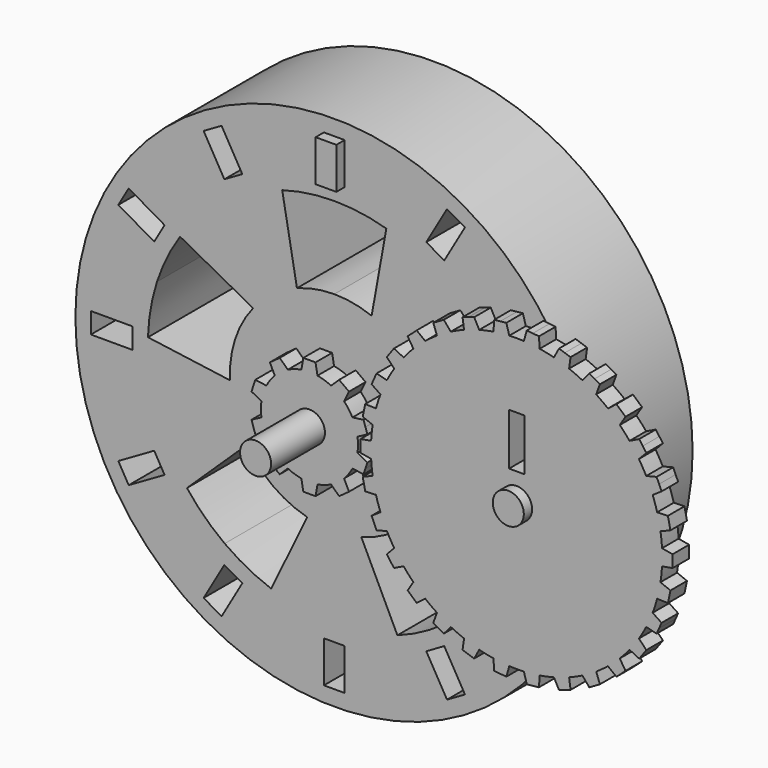
from build123d import *

# Parameters (mm, degrees)
F2_R      = 50
F3_DEPTH  = 24
F4_R      = 5
F4_R_2    = 3
F5_DEPTH  = 2
F6_DEPTH  = 19
F7_DEPTH  = 8
F12_DEPTH = 4
F14_DEPTH = 4
F15_W     = 4
F15_H     = 8
F15_W_2   = 8
F15_H_2   = 4
F16_DEPTH = 10
F17_DEPTH = 12
F19_DEPTH = 25
F20_W     = 3
F20_H     = 10
F21_DEPTH = 25


with BuildPart() as f3:
    # F2 (on Front) → F3 (new body)
    with BuildSketch(Plane.XZ):
        Circle(F2_R)
    extrude(amount=F3_DEPTH)

    # F4 (on face) → F5 (join)
    with BuildSketch(Plane.XZ.offset(24)):
        Circle(F4_R)
        Circle(F4_R_2, mode=Mode.SUBTRACT)
        with Locations((40, 0)):
            Circle(F4_R)
        with Locations((40, 0)):
            Circle(F4_R_2, mode=Mode.SUBTRACT)
    extrude(amount=F5_DEPTH)


with BuildPart() as f6:
    # F6 (new): a face of the model
    f6_faces = [f3.part.faces().sort_by_distance(p)[0] for p in [
        (0, -24, 0),
    ]]
    extrude(f6_faces, amount=F6_DEPTH)

    # F11 (on face) → F12 (join)
    with BuildSketch(Plane.XZ.offset(26)):
        with BuildLine():
            ThreePointArc((9.2729637667, -1.3794085621), (9.3494561423, -0.6915886375), (9.375, 0))
            ThreePointArc((9.375, 0), (9.3494561423, 0.6915886375), (9.2729637667, 1.3794085621))
            ThreePointArc((9.2729637667, 1.3794085621), (8.9161548403, 2.8970343223), (8.3127812852, 4.3345463782))
            ThreePointArc((8.3127812852, 4.3345463782), (7.5845343223, 5.5104867402), (6.6911892658, 6.566476316))
            ThreePointArc((6.6911892658, 6.566476316), (5.5104867402, 7.5845343223), (4.1773988938, 8.3928519278))
            ThreePointArc((4.1773988938, 8.3928519278), (2.8970343223, 8.9161548403), (1.5536078905, 9.2453733036))
            ThreePointArc((1.5536078905, 9.2453733036), (0, 9.375), (-1.5536078905, 9.2453733036))
            ThreePointArc((-1.5536078905, 9.2453733036), (-2.8970343223, 8.9161548403), (-4.1773988938, 8.3928519278))
            ThreePointArc((-4.1773988938, 8.3928519278), (-5.5104867402, 7.5845343223), (-6.6911892658, 6.566476316))
            ThreePointArc((-6.6911892658, 6.566476316), (-7.5845343223, 5.5104867402), (-8.3127812852, 4.3345463782))
            ThreePointArc((-8.3127812852, 4.3345463782), (-8.9161548403, 2.8970343223), (-9.2729637667, 1.3794085621))
            ThreePointArc((-9.2729637667, 1.3794085621), (-9.375, 0), (-9.2729637667, -1.3794085621))
            ThreePointArc((-9.2729637667, -1.3794085621), (-8.9161548403, -2.8970343223), (-8.3127812852, -4.3345463782))
            ThreePointArc((-8.3127812852, -4.3345463782), (-7.5845343223, -5.5104867402), (-6.6911892658, -6.566476316))
            ThreePointArc((-6.6911892658, -6.566476316), (-5.5104867402, -7.5845343223), (-4.1773988938, -8.3928519278))
            ThreePointArc((-4.1773988938, -8.3928519278), (-2.8970343223, -8.9161548403), (-1.5536078905, -9.2453733036))
            ThreePointArc((-1.5536078905, -9.2453733036), (0, -9.375), (1.5536078905, -9.2453733036))
            ThreePointArc((1.5536078905, -9.2453733036), (2.8970343223, -8.9161548403), (4.1773988938, -8.3928519278))
            ThreePointArc((4.1773988938, -8.3928519278), (5.5104867402, -7.5845343223), (6.6911892658, -6.566476316))
            ThreePointArc((6.6911892658, -6.566476316), (7.5845343223, -5.5104867402), (8.3127812852, -4.3345463782))
            ThreePointArc((8.3127812852, -4.3345463782), (8.9161548403, -2.8970343223), (9.2729637667, -1.3794085621))
        make_face()
        with BuildLine():
            ThreePointArc((8.3127812852, 4.3345463782), (8.9161548403, 2.8970343223), (9.2729637667, 1.3794085621))
            Line((9.2729637667, 1.3794085621), (11.1823199426, 2.3946312492))
            Line((11.1823199426, 2.3946312492), (10.8182678729, 3.515068311))
            Line((10.8182678729, 3.515068311), (10.4542158031, 4.6355053728))
            Line((10.4542158031, 4.6355053728), (8.3127812852, 4.3345463782))
        make_face()
        with BuildLine():
            Line((11.1823199426, -2.3946312492), (9.2729637667, -1.3794085621))
            ThreePointArc((9.2729637667, -1.3794085621), (8.9161548403, -2.8970343223), (8.3127812852, -4.3345463782))
            Line((8.3127812852, -4.3345463782), (10.4542158031, -4.6355053728))
            Line((10.4542158031, -4.6355053728), (10.8182678729, -3.515068311))
            Line((10.8182678729, -3.515068311), (11.1823199426, -2.3946312492))
        make_face()
        with BuildLine():
            ThreePointArc((4.1773988938, 8.3928519278), (5.5104867402, 7.5845343223), (6.6911892658, 6.566476316))
            Line((6.6911892658, 6.566476316), (7.6391579371, 8.5101001246))
            Line((7.6391579371, 8.5101001246), (6.6860572448, 9.202568311))
            Line((6.6860572448, 9.202568311), (5.7329565525, 9.8950364974))
            Line((5.7329565525, 9.8950364974), (4.1773988938, 8.3928519278))
        make_face()
        with BuildLine():
            Line((7.6391579371, -8.5101001246), (6.6911892658, -6.566476316))
            ThreePointArc((6.6911892658, -6.566476316), (5.5104867402, -7.5845343223), (4.1773988938, -8.3928519278))
            Line((4.1773988938, -8.3928519278), (5.7329565525, -9.8950364974))
            Line((5.7329565525, -9.8950364974), (6.6860572448, -9.202568311))
            Line((6.6860572448, -9.202568311), (7.6391579371, -8.5101001246))
        make_face()
        with BuildLine():
            ThreePointArc((-1.5536078905, 9.2453733036), (0, 9.375), (1.5536078905, 9.2453733036))
            Line((1.5536078905, 9.2453733036), (1.1780972451, 11.375))
            Line((1.1780972451, 11.375), (0, 11.375))
            Line((0, 11.375), (-1.1780972451, 11.375))
            Line((-1.1780972451, 11.375), (-1.5536078905, 9.2453733036))
        make_face()
        with BuildLine():
            Line((1.1780972451, -11.375), (1.5536078905, -9.2453733036))
            ThreePointArc((1.5536078905, -9.2453733036), (0, -9.375), (-1.5536078905, -9.2453733036))
            Line((-1.5536078905, -9.2453733036), (-1.1780972451, -11.375))
            Line((-1.1780972451, -11.375), (0, -11.375))
            Line((0, -11.375), (1.1780972451, -11.375))
        make_face()
        with BuildLine():
            ThreePointArc((-6.6911892658, 6.566476316), (-5.5104867402, 7.5845343223), (-4.1773988938, 8.3928519278))
            Line((-4.1773988938, 8.3928519278), (-5.7329565525, 9.8950364974))
            Line((-5.7329565525, 9.8950364974), (-6.6860572448, 9.202568311))
            Line((-6.6860572448, 9.202568311), (-7.6391579371, 8.5101001246))
            Line((-7.6391579371, 8.5101001246), (-6.6911892658, 6.566476316))
        make_face()
        with BuildLine():
            Line((-5.7329565525, -9.8950364974), (-4.1773988938, -8.3928519278))
            ThreePointArc((-4.1773988938, -8.3928519278), (-5.5104867402, -7.5845343223), (-6.6911892658, -6.566476316))
            Line((-6.6911892658, -6.566476316), (-7.6391579371, -8.5101001246))
            Line((-7.6391579371, -8.5101001246), (-6.6860572448, -9.202568311))
            Line((-6.6860572448, -9.202568311), (-5.7329565525, -9.8950364974))
        make_face()
        with BuildLine():
            ThreePointArc((-9.2729637667, 1.3794085621), (-8.9161548403, 2.8970343223), (-8.3127812852, 4.3345463782))
            Line((-8.3127812852, 4.3345463782), (-10.4542158031, 4.6355053728))
            Line((-10.4542158031, 4.6355053728), (-10.8182678729, 3.515068311))
            Line((-10.8182678729, 3.515068311), (-11.1823199426, 2.3946312492))
            Line((-11.1823199426, 2.3946312492), (-9.2729637667, 1.3794085621))
        make_face()
        with BuildLine():
            Line((-10.4542158031, -4.6355053728), (-8.3127812852, -4.3345463782))
            ThreePointArc((-8.3127812852, -4.3345463782), (-8.9161548403, -2.8970343223), (-9.2729637667, -1.3794085621))
            Line((-9.2729637667, -1.3794085621), (-11.1823199426, -2.3946312492))
            Line((-11.1823199426, -2.3946312492), (-10.8182678729, -3.515068311))
            Line((-10.8182678729, -3.515068311), (-10.4542158031, -4.6355053728))
        make_face()
    extrude(amount=F12_DEPTH)


with BuildPart() as f7:
    # F7 (new): a face of the model
    f7_faces = [f3.part.faces().sort_by_distance(p)[0] for p in [
        (40, -24, 0),
    ]]
    extrude(f7_faces, amount=F7_DEPTH)

    # F13 (on face) → F14 (join)
    with BuildSketch(Plane.XZ.offset(26)):
        with BuildLine():
            ThreePointArc((68.0829066802, -1.5381733945), (68.1144747006, -0.7693746225), (68.125, 0))
            ThreePointArc((68.125, 0), (68.1144747006, 0.7693746225), (68.0829066802, 1.5381733945))
            ThreePointArc((68.0829066802, 1.5381733945), (67.9709283072, 2.9398630294), (67.7890320221, 4.3342039956))
            ThreePointArc((67.7890320221, 4.3342039956), (67.5104012706, 5.8475163042), (67.1494235596, 7.3433252263))
            ThreePointArc((67.1494235596, 7.3433252263), (66.7484645208, 8.6911029668), (66.280643318, 10.0171558733))
            ThreePointArc((66.280643318, 10.0171558733), (65.6934659962, 11.4394680865), (65.0293803521, 12.8275385085))
            ThreePointArc((65.0293803521, 12.8275385085), (64.3569644814, 14.0625), (63.6236643925, 15.2623099717))
            ThreePointArc((63.6236643925, 15.2623099717), (62.7536029668, 16.5314602207), (61.815433119, 17.7511268046))
            ThreePointArc((61.815433119, 17.7511268046), (60.9009482166, 18.8192983038), (59.934217974, 19.8404278876))
            ThreePointArc((59.934217974, 19.8404278876), (58.8192983038, 20.9009482166), (57.6480467764, 21.8989056799))
            ThreePointArc((57.6480467764, 21.8989056799), (56.5314602207, 22.7536029668), (55.3735505752, 23.5514238999))
            ThreePointArc((55.3735505752, 23.5514238999), (54.0625, 24.3569644814), (52.709356105, 25.0895972944))
            ThreePointArc((52.709356105, 25.0895972944), (51.4394680865, 25.6934659962), (50.1409852457, 26.2331096755))
            ThreePointArc((50.1409852457, 26.2331096755), (48.6911029668, 26.7484645208), (47.2152055856, 27.1837531139))
            ThreePointArc((47.2152055856, 27.1837531139), (45.8475163042, 27.5104012706), (44.4652101991, 27.7682826779))
            ThreePointArc((44.4652101991, 27.7682826779), (42.9398630294, 27.9709283072), (41.4057159597, 28.0898484802))
            ThreePointArc((41.4057159597, 28.0898484802), (40, 28.125), (38.5942840403, 28.0898484802))
            ThreePointArc((38.5942840403, 28.0898484802), (37.0601369706, 27.9709283072), (35.5347898009, 27.7682826779))
            ThreePointArc((35.5347898009, 27.7682826779), (34.1524836958, 27.5104012706), (32.7847944144, 27.1837531139))
            ThreePointArc((32.7847944144, 27.1837531139), (31.3088970332, 26.7484645208), (29.8590147543, 26.2331096755))
            ThreePointArc((29.8590147543, 26.2331096755), (28.5605319135, 25.6934659962), (27.290643895, 25.0895972944))
            ThreePointArc((27.290643895, 25.0895972944), (25.9375, 24.3569644814), (24.6264494248, 23.5514238999))
            ThreePointArc((24.6264494248, 23.5514238999), (23.4685397793, 22.7536029668), (22.3519532236, 21.8989056799))
            ThreePointArc((22.3519532236, 21.8989056799), (21.1807016962, 20.9009482166), (20.065782026, 19.8404278876))
            ThreePointArc((20.065782026, 19.8404278876), (19.0990517834, 18.8192983038), (18.184566881, 17.7511268046))
            ThreePointArc((18.184566881, 17.7511268046), (17.2463970332, 16.5314602207), (16.3763356075, 15.2623099717))
            ThreePointArc((16.3763356075, 15.2623099717), (15.6430355186, 14.0625), (14.9706196479, 12.8275385085))
            ThreePointArc((14.9706196479, 12.8275385085), (14.3065340038, 11.4394680865), (13.719356682, 10.0171558733))
            ThreePointArc((13.719356682, 10.0171558733), (13.2515354792, 8.6911029668), (12.8505764404, 7.3433252263))
            ThreePointArc((12.8505764404, 7.3433252263), (12.4895987294, 5.8475163042), (12.2109679779, 4.3342039956))
            ThreePointArc((12.2109679779, 4.3342039956), (12.0290716928, 2.9398630294), (11.9170933198, 1.5381733945))
            ThreePointArc((11.9170933198, 1.5381733945), (11.875, 0), (11.9170933198, -1.5381733945))
            ThreePointArc((11.9170933198, -1.5381733945), (12.0290716928, -2.9398630294), (12.2109679779, -4.3342039956))
            ThreePointArc((12.2109679779, -4.3342039956), (12.4895987294, -5.8475163042), (12.8505764404, -7.3433252263))
            ThreePointArc((12.8505764404, -7.3433252263), (13.2515354792, -8.6911029668), (13.719356682, -10.0171558733))
            ThreePointArc((13.719356682, -10.0171558733), (14.3065340038, -11.4394680865), (14.9706196479, -12.8275385085))
            ThreePointArc((14.9706196479, -12.8275385085), (15.6430355186, -14.0625), (16.3763356075, -15.2623099717))
            ThreePointArc((16.3763356075, -15.2623099717), (17.2463970332, -16.5314602207), (18.184566881, -17.7511268046))
            ThreePointArc((18.184566881, -17.7511268046), (19.0990517834, -18.8192983038), (20.065782026, -19.8404278876))
            ThreePointArc((20.065782026, -19.8404278876), (21.1807016962, -20.9009482166), (22.3519532236, -21.8989056799))
            ThreePointArc((22.3519532236, -21.8989056799), (23.4685397793, -22.7536029668), (24.6264494248, -23.5514238999))
            ThreePointArc((24.6264494248, -23.5514238999), (25.9375, -24.3569644814), (27.290643895, -25.0895972944))
            ThreePointArc((27.290643895, -25.0895972944), (28.5605319135, -25.6934659962), (29.8590147543, -26.2331096755))
            ThreePointArc((29.8590147543, -26.2331096755), (31.3088970332, -26.7484645208), (32.7847944144, -27.1837531139))
            ThreePointArc((32.7847944144, -27.1837531139), (34.1524836958, -27.5104012706), (35.5347898009, -27.7682826779))
            ThreePointArc((35.5347898009, -27.7682826779), (37.0601369706, -27.9709283072), (38.5942840403, -28.0898484802))
            ThreePointArc((38.5942840403, -28.0898484802), (40, -28.125), (41.4057159597, -28.0898484802))
            ThreePointArc((41.4057159597, -28.0898484802), (42.9398630294, -27.9709283072), (44.4652101991, -27.7682826779))
            ThreePointArc((44.4652101991, -27.7682826779), (45.8475163042, -27.5104012706), (47.2152055856, -27.1837531139))
            ThreePointArc((47.2152055856, -27.1837531139), (48.6911029668, -26.7484645208), (50.1409852457, -26.2331096755))
            ThreePointArc((50.1409852457, -26.2331096755), (51.4394680865, -25.6934659962), (52.709356105, -25.0895972944))
            ThreePointArc((52.709356105, -25.0895972944), (54.0625, -24.3569644814), (55.3735505752, -23.5514238999))
            ThreePointArc((55.3735505752, -23.5514238999), (56.5314602207, -22.7536029668), (57.6480467764, -21.8989056799))
            ThreePointArc((57.6480467764, -21.8989056799), (58.8192983038, -20.9009482166), (59.934217974, -19.8404278876))
            ThreePointArc((59.934217974, -19.8404278876), (60.9009482166, -18.8192983038), (61.815433119, -17.7511268046))
            ThreePointArc((61.815433119, -17.7511268046), (62.7536029668, -16.5314602207), (63.6236643925, -15.2623099717))
            ThreePointArc((63.6236643925, -15.2623099717), (64.3569644814, -14.0625), (65.0293803521, -12.8275385085))
            ThreePointArc((65.0293803521, -12.8275385085), (65.6934659962, -11.4394680865), (66.280643318, -10.0171558733))
            ThreePointArc((66.280643318, -10.0171558733), (66.7484645208, -8.6911029668), (67.1494235596, -7.3433252263))
            ThreePointArc((67.1494235596, -7.3433252263), (67.5104012706, -5.8475163042), (67.7890320221, -4.3342039956))
            ThreePointArc((67.7890320221, -4.3342039956), (67.9709283072, -2.9398630294), (68.0829066802, -1.5381733945))
        make_face()
        with BuildLine():
            ThreePointArc((68.0829066802, 1.5381733945), (68.1144747006, 0.7693746225), (68.125, 0))
            ThreePointArc((68.125, 0), (68.1144747006, -0.7693746225), (68.0829066802, -1.5381733945))
            Line((68.0829066802, -1.5381733945), (70.125, -1.1780972451))
            Line((70.125, -1.1780972451), (70.125, 0))
            Line((70.125, 0), (70.125, 1.1780972451))
            Line((70.125, 1.1780972451), (68.0829066802, 1.5381733945))
        make_face()
        with BuildLine():
            ThreePointArc((67.1494235596, 7.3433252263), (67.5104012706, 5.8475163042), (67.7890320221, 4.3342039956))
            Line((67.7890320221, 4.3342039956), (69.7116366623, 5.1109866922))
            Line((69.7116366623, 5.1109866922), (69.4666964721, 6.2633396859))
            Line((69.4666964721, 6.2633396859), (69.2217562819, 7.4156926796))
            Line((69.2217562819, 7.4156926796), (67.1494235596, 7.3433252263))
        make_face()
        with BuildLine():
            Line((69.7116366623, -5.1109866922), (67.7890320221, -4.3342039956))
            ThreePointArc((67.7890320221, -4.3342039956), (67.5104012706, -5.8475163042), (67.1494235596, -7.3433252263))
            Line((67.1494235596, -7.3433252263), (69.2217562819, -7.4156926796))
            Line((69.2217562819, -7.4156926796), (69.4666964721, -6.2633396859))
            Line((69.4666964721, -6.2633396859), (69.7116366623, -5.1109866922))
        make_face()
        with BuildLine():
            ThreePointArc((65.0293803521, 12.8275385085), (65.6934659962, 11.4394680865), (66.280643318, 10.0171558733))
            Line((66.280643318, 10.0171558733), (67.9997322302, 11.1766959857))
            Line((67.9997322302, 11.1766959857), (67.5205569115, 12.2529413727))
            Line((67.5205569115, 12.2529413727), (67.0413815928, 13.3291867596))
            Line((67.0413815928, 13.3291867596), (65.0293803521, 12.8275385085))
        make_face()
        with BuildLine():
            Line((67.9997322302, -11.1766959857), (66.280643318, -10.0171558733))
            ThreePointArc((66.280643318, -10.0171558733), (65.6934659962, -11.4394680865), (65.0293803521, -12.8275385085))
            Line((65.0293803521, -12.8275385085), (67.0413815928, -13.3291867596))
            Line((67.0413815928, -13.3291867596), (67.5205569115, -12.2529413727))
            Line((67.5205569115, -12.2529413727), (67.9997322302, -11.1766959857))
        make_face()
        with BuildLine():
            ThreePointArc((61.815433119, 17.7511268046), (62.7536029668, 16.5314602207), (63.6236643925, 15.2623099717))
            Line((63.6236643925, 15.2623099717), (65.064105142, 16.753930033))
            Line((65.064105142, 16.753930033), (64.3716369555, 17.7070307253))
            Line((64.3716369555, 17.7070307253), (63.6791687691, 18.6601314176))
            Line((63.6791687691, 18.6601314176), (61.815433119, 17.7511268046))
        make_face()
        with BuildLine():
            Line((65.064105142, -16.753930033), (63.6236643925, -15.2623099717))
            ThreePointArc((63.6236643925, -15.2623099717), (62.7536029668, -16.5314602207), (61.815433119, -17.7511268046))
            Line((61.815433119, -17.7511268046), (63.6791687691, -18.6601314176))
            Line((63.6791687691, -18.6601314176), (64.3716369555, -17.7070307253))
            Line((64.3716369555, -17.7070307253), (65.064105142, -16.753930033))
        make_face()
        with BuildLine():
            ThreePointArc((57.6480467764, 21.8989056799), (58.8192983038, 20.9009482166), (59.934217974, 19.8404278876))
            Line((59.934217974, 19.8404278876), (61.0330563882, 21.5989369435))
            Line((61.0330563882, 21.5989369435), (60.1575595166, 22.3872378675))
            Line((60.1575595166, 22.3872378675), (59.282062645, 23.1755387915))
            Line((59.282062645, 23.1755387915), (57.6480467764, 21.8989056799))
        make_face()
        with BuildLine():
            Line((61.0330563882, -21.5989369435), (59.934217974, -19.8404278876))
            ThreePointArc((59.934217974, -19.8404278876), (58.8192983038, -20.9009482166), (57.6480467764, -21.8989056799))
            Line((57.6480467764, -21.8989056799), (59.282062645, -23.1755387915))
            Line((59.282062645, -23.1755387915), (60.1575595166, -22.3872378675))
            Line((60.1575595166, -22.3872378675), (61.0330563882, -21.5989369435))
        make_face()
        with BuildLine():
            ThreePointArc((52.709356105, 25.0895972944), (54.0625, 24.3569644814), (55.3735505752, 23.5514238999))
            Line((55.3735505752, 23.5514238999), (56.0827621424, 25.4999666665))
            Line((56.0827621424, 25.4999666665), (55.0625, 26.089015289))
            Line((55.0625, 26.089015289), (54.0422378576, 26.6780639116))
            Line((54.0422378576, 26.6780639116), (52.709356105, 25.0895972944))
        make_face()
        with BuildLine():
            Line((56.0827621424, -25.4999666665), (55.3735505752, -23.5514238999))
            ThreePointArc((55.3735505752, -23.5514238999), (54.0625, -24.3569644814), (52.709356105, -25.0895972944))
            Line((52.709356105, -25.0895972944), (54.0422378576, -26.6780639116))
            Line((54.0422378576, -26.6780639116), (55.0625, -26.089015289))
            Line((55.0625, -26.089015289), (56.0827621424, -25.4999666665))
        make_face()
        with BuildLine():
            ThreePointArc((47.2152055856, 27.1837531139), (48.6911029668, 26.7484645208), (50.1409852457, 26.2331096755))
            Line((50.1409852457, 26.2331096755), (50.4295740173, 28.2865254836))
            Line((50.4295740173, 28.2865254836), (49.3091369555, 28.6505775534))
            Line((49.3091369555, 28.6505775534), (48.1886998938, 29.0146296232))
            Line((48.1886998938, 29.0146296232), (47.2152055856, 27.1837531139))
        make_face()
        with BuildLine():
            Line((50.4295740173, -28.2865254836), (50.1409852457, -26.2331096755))
            ThreePointArc((50.1409852457, -26.2331096755), (48.6911029668, -26.7484645208), (47.2152055856, -27.1837531139))
            Line((47.2152055856, -27.1837531139), (48.1886998938, -29.0146296232))
            Line((48.1886998938, -29.0146296232), (49.3091369555, -28.6505775534))
            Line((49.3091369555, -28.6505775534), (50.4295740173, -28.2865254836))
        make_face()
        with BuildLine():
            ThreePointArc((41.4057159597, 28.0898484802), (42.9398630294, 27.9709283072), (44.4652101991, 27.7682826779))
            Line((44.4652101991, 27.7682826779), (44.3205634611, 29.8368274034))
            Line((44.3205634611, 29.8368274034), (43.1489199559, 29.959972098))
            Line((43.1489199559, 29.959972098), (41.9772764508, 30.0831167926))
            Line((41.9772764508, 30.0831167926), (41.4057159597, 28.0898484802))
        make_face()
        with BuildLine():
            Line((44.3205634611, -29.8368274034), (44.4652101991, -27.7682826779))
            ThreePointArc((44.4652101991, -27.7682826779), (42.9398630294, -27.9709283072), (41.4057159597, -28.0898484802))
            Line((41.4057159597, -28.0898484802), (41.9772764508, -30.0831167926))
            Line((41.9772764508, -30.0831167926), (43.1489199559, -29.959972098))
            Line((43.1489199559, -29.959972098), (44.3205634611, -29.8368274034))
        make_face()
        with BuildLine():
            ThreePointArc((35.5347898009, 27.7682826779), (37.0601369706, 27.9709283072), (38.5942840403, 28.0898484802))
            Line((38.5942840403, 28.0898484802), (38.0227235492, 30.0831167926))
            Line((38.0227235492, 30.0831167926), (36.8510800441, 29.959972098))
            Line((36.8510800441, 29.959972098), (35.6794365389, 29.8368274034))
            Line((35.6794365389, 29.8368274034), (35.5347898009, 27.7682826779))
        make_face()
        with BuildLine():
            Line((38.0227235492, -30.0831167926), (38.5942840403, -28.0898484802))
            ThreePointArc((38.5942840403, -28.0898484802), (37.0601369706, -27.9709283072), (35.5347898009, -27.7682826779))
            Line((35.5347898009, -27.7682826779), (35.6794365389, -29.8368274034))
            Line((35.6794365389, -29.8368274034), (36.8510800441, -29.959972098))
            Line((36.8510800441, -29.959972098), (38.0227235492, -30.0831167926))
        make_face()
        with BuildLine():
            ThreePointArc((29.8590147543, 26.2331096755), (31.3088970332, 26.7484645208), (32.7847944144, 27.1837531139))
            Line((32.7847944144, 27.1837531139), (31.8113001062, 29.0146296232))
            Line((31.8113001062, 29.0146296232), (30.6908630445, 28.6505775534))
            Line((30.6908630445, 28.6505775534), (29.5704259827, 28.2865254836))
            Line((29.5704259827, 28.2865254836), (29.8590147543, 26.2331096755))
        make_face()
        with BuildLine():
            Line((31.8113001062, -29.0146296232), (32.7847944144, -27.1837531139))
            ThreePointArc((32.7847944144, -27.1837531139), (31.3088970332, -26.7484645208), (29.8590147543, -26.2331096755))
            Line((29.8590147543, -26.2331096755), (29.5704259827, -28.2865254836))
            Line((29.5704259827, -28.2865254836), (30.6908630445, -28.6505775534))
            Line((30.6908630445, -28.6505775534), (31.8113001062, -29.0146296232))
        make_face()
        with BuildLine():
            ThreePointArc((24.6264494248, 23.5514238999), (25.9375, 24.3569644814), (27.290643895, 25.0895972944))
            Line((27.290643895, 25.0895972944), (25.9577621424, 26.6780639116))
            Line((25.9577621424, 26.6780639116), (24.9375, 26.089015289))
            Line((24.9375, 26.089015289), (23.9172378576, 25.4999666665))
            Line((23.9172378576, 25.4999666665), (24.6264494248, 23.5514238999))
        make_face()
        with BuildLine():
            Line((25.9577621424, -26.6780639116), (27.290643895, -25.0895972944))
            ThreePointArc((27.290643895, -25.0895972944), (25.9375, -24.3569644814), (24.6264494248, -23.5514238999))
            Line((24.6264494248, -23.5514238999), (23.9172378576, -25.4999666665))
            Line((23.9172378576, -25.4999666665), (24.9375, -26.089015289))
            Line((24.9375, -26.089015289), (25.9577621424, -26.6780639116))
        make_face()
        with BuildLine():
            ThreePointArc((20.065782026, 19.8404278876), (21.1807016962, 20.9009482166), (22.3519532236, 21.8989056799))
            Line((22.3519532236, 21.8989056799), (20.717937355, 23.1755387915))
            Line((20.717937355, 23.1755387915), (19.8424404834, 22.3872378675))
            Line((19.8424404834, 22.3872378675), (18.9669436118, 21.5989369435))
            Line((18.9669436118, 21.5989369435), (20.065782026, 19.8404278876))
        make_face()
        with BuildLine():
            Line((20.717937355, -23.1755387915), (22.3519532236, -21.8989056799))
            ThreePointArc((22.3519532236, -21.8989056799), (21.1807016962, -20.9009482166), (20.065782026, -19.8404278876))
            Line((20.065782026, -19.8404278876), (18.9669436118, -21.5989369435))
            Line((18.9669436118, -21.5989369435), (19.8424404834, -22.3872378675))
            Line((19.8424404834, -22.3872378675), (20.717937355, -23.1755387915))
        make_face()
        with BuildLine():
            ThreePointArc((16.3763356075, 15.2623099717), (17.2463970332, 16.5314602207), (18.184566881, 17.7511268046))
            Line((18.184566881, 17.7511268046), (16.3208312309, 18.6601314176))
            Line((16.3208312309, 18.6601314176), (15.6283630445, 17.7070307253))
            Line((15.6283630445, 17.7070307253), (14.935894858, 16.753930033))
            Line((14.935894858, 16.753930033), (16.3763356075, 15.2623099717))
        make_face()
        with BuildLine():
            Line((16.3208312309, -18.6601314176), (18.184566881, -17.7511268046))
            ThreePointArc((18.184566881, -17.7511268046), (17.2463970332, -16.5314602207), (16.3763356075, -15.2623099717))
            Line((16.3763356075, -15.2623099717), (14.935894858, -16.753930033))
            Line((14.935894858, -16.753930033), (15.6283630445, -17.7070307253))
            Line((15.6283630445, -17.7070307253), (16.3208312309, -18.6601314176))
        make_face()
        with BuildLine():
            ThreePointArc((13.719356682, 10.0171558733), (14.3065340038, 11.4394680865), (14.9706196479, 12.8275385085))
            Line((14.9706196479, 12.8275385085), (12.9586184072, 13.3291867596))
            Line((12.9586184072, 13.3291867596), (12.4794430885, 12.2529413727))
            Line((12.4794430885, 12.2529413727), (12.0002677698, 11.1766959857))
            Line((12.0002677698, 11.1766959857), (13.719356682, 10.0171558733))
        make_face()
        with BuildLine():
            Line((12.9586184072, -13.3291867596), (14.9706196479, -12.8275385085))
            ThreePointArc((14.9706196479, -12.8275385085), (14.3065340038, -11.4394680865), (13.719356682, -10.0171558733))
            Line((13.719356682, -10.0171558733), (12.0002677698, -11.1766959857))
            Line((12.0002677698, -11.1766959857), (12.4794430885, -12.2529413727))
            Line((12.4794430885, -12.2529413727), (12.9586184072, -13.3291867596))
        make_face()
        with BuildLine():
            ThreePointArc((12.2109679779, 4.3342039956), (12.4895987294, 5.8475163042), (12.8505764404, 7.3433252263))
            Line((12.8505764404, 7.3433252263), (10.7782437181, 7.4156926796))
            Line((10.7782437181, 7.4156926796), (10.5333035279, 6.2633396859))
            Line((10.5333035279, 6.2633396859), (10.2883633377, 5.1109866922))
            Line((10.2883633377, 5.1109866922), (12.2109679779, 4.3342039956))
        make_face()
        with BuildLine():
            Line((10.7782437181, -7.4156926796), (12.8505764404, -7.3433252263))
            ThreePointArc((12.8505764404, -7.3433252263), (12.4895987294, -5.8475163042), (12.2109679779, -4.3342039956))
            Line((12.2109679779, -4.3342039956), (10.2883633377, -5.1109866922))
            Line((10.2883633377, -5.1109866922), (10.5333035279, -6.2633396859))
            Line((10.5333035279, -6.2633396859), (10.7782437181, -7.4156926796))
        make_face()
        with BuildLine():
            ThreePointArc((11.9170933198, -1.5381733945), (11.875, 0), (11.9170933198, 1.5381733945))
            Line((11.9170933198, 1.5381733945), (9.875, 1.1780972451))
            Line((9.875, 1.1780972451), (9.875, 0))
            Line((9.875, 0), (9.875, -1.1780972451))
            Line((9.875, -1.1780972451), (11.9170933198, -1.5381733945))
        make_face()
    extrude(amount=F14_DEPTH)

    # F20 (on face) → F21 (cut)
    with BuildSketch(Plane.XZ.offset(30)):
        with Locations((40.0521658097, 10.4745347053)):
            Rectangle(F20_W, F20_H)
    extrude(amount=-F21_DEPTH, mode=Mode.SUBTRACT)


with BuildPart() as f3_1:
    add(f3.part)

    # F15 (on face) → F16 (cut)
    with BuildSketch(Plane.XZ.offset(24)):
        with Locations((0, 43)):
            Rectangle(F15_W, F15_H)
        Polygon((-17.7679491924, 34.7749907476), (-21.7679491924, 41.7031939779), (-25.2320508076, 39.7031939779), (-21.2320508076, 32.7749907476), align=None)
        Polygon((-32.7749907476, 21.2320508076), (-39.7031939779, 25.2320508076), (-41.7031939779, 21.7679491924), (-34.7749907476, 17.7679491924), align=None)
        with Locations((-43, 0)):
            Rectangle(F15_W_2, F15_H_2)
        Polygon((-34.7749907476, -17.7679491924), (-41.7031939779, -21.7679491924), (-39.7031939779, -25.2320508076), (-32.7749907476, -21.2320508076), align=None)
        Polygon((-21.2320508076, -32.7749907476), (-25.2320508076, -39.7031939779), (-21.7679491924, -41.7031939779), (-17.7679491924, -34.7749907476), align=None)
        with Locations((0, -43)):
            Rectangle(F15_W, F15_H)
        Polygon((17.7679491924, -34.7749907476), (21.7679491924, -41.7031939779), (25.2320508076, -39.7031939779), (21.2320508076, -32.7749907476), align=None)
        Polygon((32.7749907476, -21.2320508076), (39.7031939779, -25.2320508076), (41.7031939779, -21.7679491924), (34.7749907476, -17.7679491924), align=None)
        with Locations((43, 0)):
            Rectangle(F15_W_2, F15_H_2)
        Polygon((34.7749907476, 17.7679491924), (41.7031939779, 21.7679491924), (39.7031939779, 25.2320508076), (32.7749907476, 21.2320508076), align=None)
        Polygon((21.2320508076, 32.7749907476), (25.2320508076, 39.7031939779), (21.7679491924, 41.7031939779), (17.7679491924, 34.7749907476), align=None)
    extrude(amount=-F16_DEPTH, mode=Mode.SUBTRACT)


with BuildPart() as f17:
    # F17 (new): a face of the model
    f17_faces = [f3_1.part.faces().sort_by_distance(p)[0] for p in [
        (0, -14, 43),
    ]]
    extrude(f17_faces, amount=F17_DEPTH)


with BuildPart() as f3_2:
    add(f3_1.part)

    # F18 (on face) → F19 (cut)
    with BuildSketch(Plane.XZ.offset(24)):
        with BuildLine():
            Line((-10.0523579749, 34.5680502653), (-7.2116198146, 18.8222506126))
            ThreePointArc((-7.2116198146, 18.8222506126), (-3.667004482, 19.820132608), (0, 20.1565021388))
            ThreePointArc((0, 20.1565021388), (3.667004482, 19.820132608), (7.2116198146, 18.8222506126))
            Line((7.2116198146, 18.8222506126), (10.0523579749, 34.5680502653))
            ThreePointArc((10.0523579749, 34.5680502653), (5.0769178863, 35.6402147128), (0, 36))
            ThreePointArc((0, 36), (-5.0769178863, 35.6402147128), (-10.0523579749, 34.5680502653))
        make_face()
        with BuildLine():
            ThreePointArc((-34.2380345866, 11.1246117975), (-35.4647123507, 6.184996191), (-35.9825189082, 1.1217544383))
            Line((-35.9825189082, 1.1217544383), (-20.1295371761, -1.042262706))
            ThreePointArc((-20.1295371761, -1.042262706), (-19.9832329741, 2.6372292987), (-19.1699727048, 6.228701708))
            ThreePointArc((-19.1699727048, 6.228701708), (-17.7168995673, 9.6122863146), (-15.6725110167, 12.6750533294))
            Line((-15.6725110167, 12.6750533294), (-29.7698200127, 20.2424755505))
            ThreePointArc((-29.7698200127, 20.2424755505), (-32.3270045389, 15.8418678679), (-34.2380345866, 11.1246117975))
        make_face()
        with BuildLine():
            ThreePointArc((-21.1602690825, -29.1246117975), (-16.8414797477, -31.8176768465), (-12.1860617112, -33.8747678954))
            Line((-12.1860617112, -33.8747678954), (-5.229118338, -19.4664043901))
            ThreePointArc((-5.229118338, -19.4664043901), (-8.6833127011, -18.1902352653), (-11.847694695, -16.3069527775))
            ThreePointArc((-11.847694695, -16.3069527775), (-14.6166505899, -13.879412956), (-16.897764312, -10.9886368458))
            Line((-16.897764312, -10.9886368458), (-28.4511185817, -22.0575123586))
            ThreePointArc((-28.4511185817, -22.0575123586), (-25.0561054458, -25.8494019252), (-21.1602690825, -29.1246117975))
        make_face()
        with BuildLine():
            ThreePointArc((21.1602690825, -29.1246117975), (25.0561054458, -25.8494019252), (28.4511185817, -22.0575123586))
            Line((28.4511185817, -22.0575123586), (16.897764312, -10.9886368458))
            ThreePointArc((16.897764312, -10.9886368458), (14.6166505899, -13.879412956), (11.847694695, -16.3069527775))
            ThreePointArc((11.847694695, -16.3069527775), (8.6833127011, -18.1902352653), (5.229118338, -19.4664043901))
            Line((5.229118338, -19.4664043901), (12.1860617112, -33.8747678954))
            ThreePointArc((12.1860617112, -33.8747678954), (16.8414797477, -31.8176768465), (21.1602690825, -29.1246117975))
        make_face()
        with BuildLine():
            ThreePointArc((34.2380345866, 11.1246117975), (32.3270045389, 15.8418678679), (29.7698200127, 20.2424755505))
            Line((29.7698200127, 20.2424755505), (15.6725110167, 12.6750533294))
            ThreePointArc((15.6725110167, 12.6750533294), (17.7168995673, 9.6122863146), (19.1699727048, 6.228701708))
            ThreePointArc((19.1699727048, 6.228701708), (19.9832329741, 2.6372292987), (20.1295371761, -1.042262706))
            Line((20.1295371761, -1.042262706), (35.9825189082, 1.1217544383))
            ThreePointArc((35.9825189082, 1.1217544383), (35.4647123507, 6.184996191), (34.2380345866, 11.1246117975))
        make_face()
    extrude(amount=-F19_DEPTH, mode=Mode.SUBTRACT)


solid = Compound([f6.part, f7.part, f17.part, f3_2.part])
